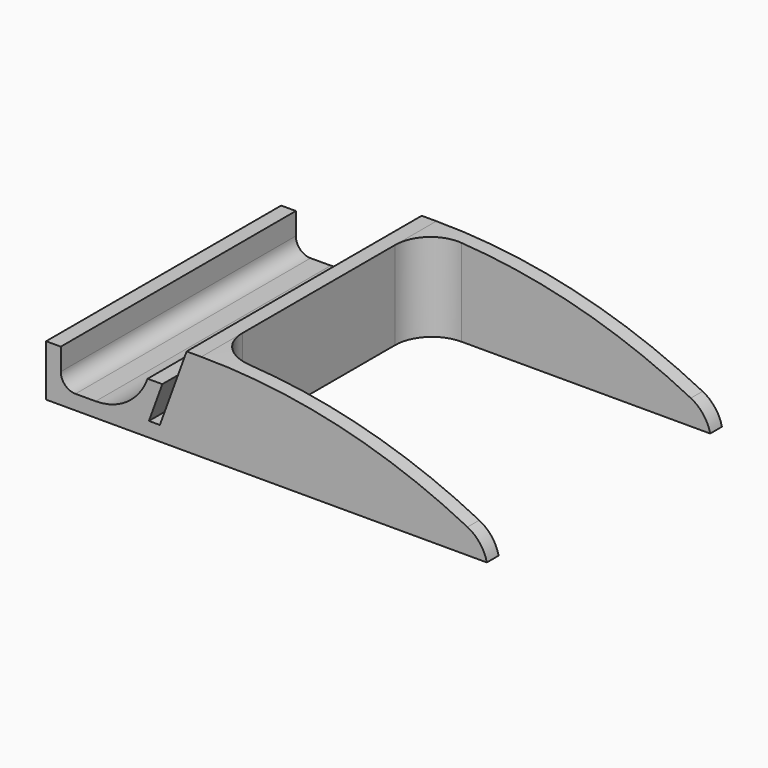
from build123d import *

# Parameters (mm, degrees)
F1_DEPTH    = 40
F2_W        = 38.8704487759
F2_H        = 36
F3_DEPTH    = 25
F4_R        = 7.5
F5_R        = 2
F6_T1_DEPTH = 16.8824680596
F6_T3_DEPTH = 16.8824680596
F7_R        = 5


# Not quite as in the source:
# - a fillet or chamfer that OpenCascade refuses, or shapes differently, is made with other operations: its cross-section is extruded or revolved along the edge and cut away or added


with BuildPart() as f1:
    # F0 (on Front) → F1 (new body)
    with BuildSketch(Plane.XZ):
        with BuildLine():
            Line((-48, 0), (-58, 0))
            Line((-58, 0), (-58, 5))
            Line((-58, 5), (-60, 5))
            Line((-60, 5), (-60, -2))
            Line((-60, -2), (0, -2))
            Line((0, -2), (0, 0))
            ThreePointArc((0, 0), (-18.8023659823, 7.4599490238), (-38.8704487759, 10))
            Line((-38.8704487759, 10), (-40.8704487759, 10))
            Line((-40.8704487759, 10), (-44.5101511185, 0))
            Line((-44.5101511185, 0), (-46, 0))
            Line((-46, 0), (-44.1801488287, 5))
            Line((-44.1801488287, 5), (-46.1801488287, 5))
            Line((-46.1801488287, 5), (-48, 0))
        make_face()
    extrude(amount=F1_DEPTH)

    # F2 (on face) → F3 (cut)
    with BuildSketch(Plane.XY.offset(10)):
        with Locations((-19.4352243879, -20)):
            Rectangle(F2_W, F2_H)
    extrude(amount=-F3_DEPTH, mode=Mode.SUBTRACT)

    # F4
    f4_edges = [f1.edges().sort_by_distance(p)[0] for p in [
        (-48, -20, 0),
    ]]
    fillet(f4_edges, radius=F4_R)

    # F5
    f5_edges = [f1.edges().sort_by_distance(p)[0] for p in [
        (-58, -20, 0),
    ]]
    fillet(f5_edges, radius=F5_R)

    # F6: fillet of radius 5 on 2 edges, made by hand

    # F6_s2 → F6_t1 (cut)
    with BuildSketch(Plane.XZ.offset(30.5587659702)):
        with BuildLine():
            ThreePointArc((0, -2), (-0.9346139409, -0.0091871804), (-2.6330480047, 1.3880102401))
            ThreePointArc((-2.6330480047, 1.3880102401), (-1.3101118631, 0.7061689139), (0, 0))
            Line((0, 0), (0, -2))
        make_face()
    extrude(amount=F6_T1_DEPTH, mode=Mode.SUBTRACT)

    # F6_s4 → F6_t3 (cut)
    with BuildSketch(Plane.XZ.offset(-7.4412340298)):
        with BuildLine():
            ThreePointArc((0, -2), (-0.9346139409, -0.0091871804), (-2.6330480047, 1.3880102401))
            ThreePointArc((-2.6330480047, 1.3880102401), (-1.3101118631, 0.7061689139), (0, 0))
            Line((0, 0), (0, -2))
        make_face()
    extrude(amount=F6_T3_DEPTH, mode=Mode.SUBTRACT)

    # F7
    f7_edges = [f1.edges().sort_by_distance(p)[0] for p in [
        (-38.870449, -38, 4),
        (-38.870449, -2, 4),
    ]]
    fillet(f7_edges, radius=F7_R)


solid = f1.part
